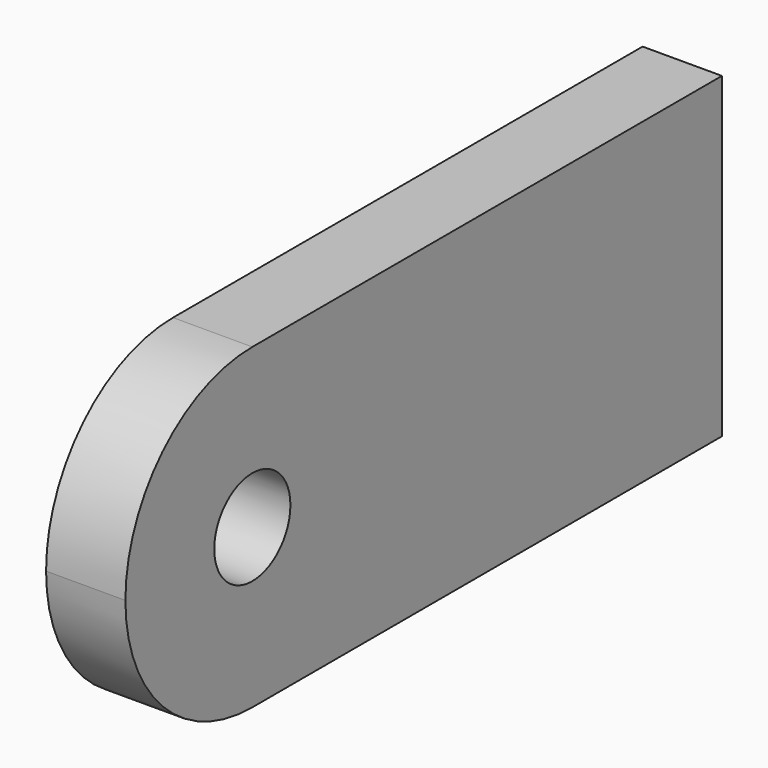
from build123d import *

# Parameters (mm, degrees)
F0_W     = 235
F0_H     = 100
F0_R     = 15
F1_DEPTH = 25
F2_R     = 49.99999


# Not quite as in the source:
# - a fillet or chamfer is up to 0.001 mm smaller than in the source, because OpenCascade refuses the exact size


with BuildPart() as f1:
    # F0 (on Right) → F1 (new body)
    with BuildSketch(Plane.YZ):
        with Locations((67.5, 0)):
            Rectangle(F0_W, F0_H)
        Circle(F0_R, mode=Mode.SUBTRACT)
    extrude(amount=F1_DEPTH)

    # F2 (radius 50 in the source; OpenCascade refuses exactly that, so slightly less here)
    f2_edges = [f1.edges().sort_by_distance(p)[0] for p in [
        (12.5, -50, 50),
        (12.5, -50, -50),
    ]]
    fillet(f2_edges, radius=F2_R)


solid = f1.part
